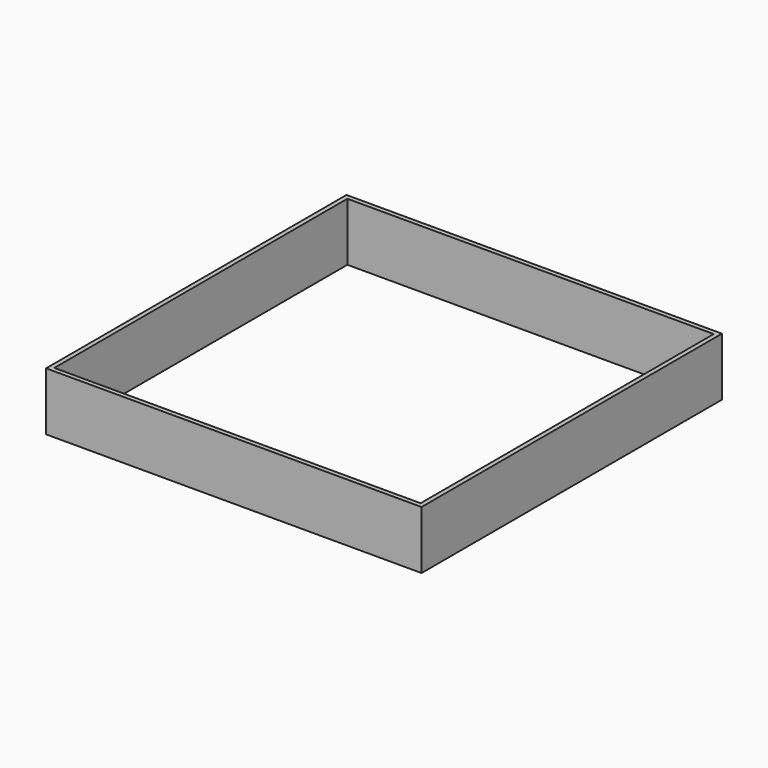
from build123d import *

# Parameters (mm, degrees)
F0_W     = 41
F0_H     = 41
F0_W_2   = 40
F0_H_2   = 40
F1_DEPTH = 6.35


# Not quite as in the source:
# - the program builds the solid bodies; features that only make, move or delete a surface that nothing else refers to are left out


with BuildPart() as f1:
    # F0 (on Top) → F1 (new body)
    with BuildSketch(Plane.XY):
        Rectangle(F0_W, F0_H)
        Rectangle(F0_W_2, F0_H_2, mode=Mode.SUBTRACT)
    extrude(amount=F1_DEPTH)


solid = f1.part
